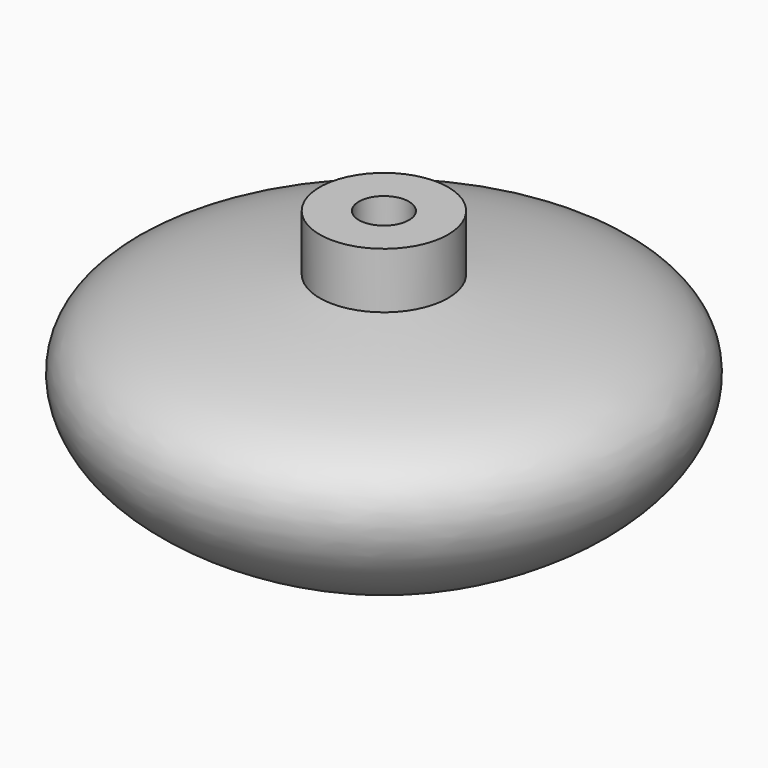
from build123d import *

# Parameters (mm, degrees)
F3_D     = 9.906
F3_DEPTH = 9.525
F3_TIP   = 2.976062646


with BuildPart() as f1:
    # F0 (on Front) → F1 (revolve)
    with BuildSketch(Plane.XZ):
        with BuildLine():
            Line((0, 63.5), (0, 0))
            add(Edge.make_bspline(
                [(0, 0), (20.0810124413, 7.472930486), (51.505453427, 19.1831941683), (54.6300398828, 47.6353373564), (28.089994696, 50.5706208252), (12.7, 52.4410080066)],
                knots=[0, 0, 0, 0, 0.4175312333, 0.6493837023, 1, 1, 1, 1], degree=3))
            Line((12.7, 52.4410080066), (12.7, 63.5))
            Line((12.7, 63.5), (0, 63.5))
        make_face()
    revolve(axis=Axis((0, 0, 31.75), (0, 0, -1)))

    # F3
    with Locations(Plane.XY.offset(63.5)):
        with Locations((0, 0)):
            Hole(F3_D / 2, depth=F3_DEPTH)
            with Locations((0, 0, -(F3_DEPTH + F3_TIP / 2))):  # 118° drill point
                Cone(0, F3_D / 2, F3_TIP, mode=Mode.SUBTRACT)


solid = f1.part
